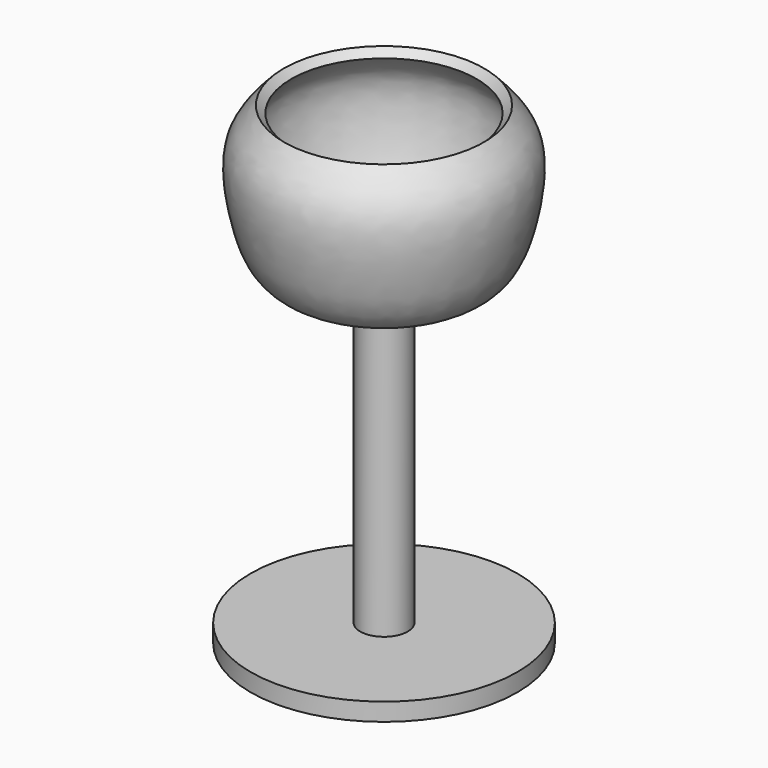
from build123d import *


# Not quite as in the source:
# - the dataset's text gives a spline's control points without its knots; the knots are read off the source's solid


with BuildPart() as f1:
    # F0 (on Front) → F1 (revolve)
    with BuildSketch(Plane.XZ):
        with BuildLine():
            Line((-33.3114092118, -56.5219796077), (-3.3958540803, -56.5219796077))
            Line((-3.3958540803, -56.5219796077), (-3.3958540803, -52.0700030029))
            Line((-3.3958540803, -52.0700030029), (-3.3958540803, 17.4802527591))
            add(Edge.make_bspline(
                [(-3.3958540803, 17.4802527591), (-3.3958541705, 17.9874718655), (-3.4894182694, 18.9850607329), (-3.9552971661, 20.3950614541), (-4.7364240353, 21.6166062828), (-5.730456479, 22.5691381333), (-6.824989545, 23.2653337421), (-7.9612562833, 23.7659449911), (-9.1199618827, 24.1286972097), (-10.6872079124, 24.4847423795), (-12.6794090241, 24.7690811344), (-15.057700209, 25.020810082), (-16.9353054891, 25.2572720748), (-18.3004868031, 25.5091381546), (-19.0782015912, 25.6983898999), (-19.6453651181, 25.8706576014), (-20.1689159088, 26.0552640278), (-21.0237206953, 26.4289307261), (-22.0986256248, 27.1000061621), (-23.2231720549, 28.1270764831), (-24.2169952979, 29.3842127548), (-25.0906025524, 30.8622732772), (-25.8487547346, 32.5336407625), (-26.499795979, 34.3600080021), (-27.0576108529, 36.2980435215), (-27.4605598647, 37.9723758628), (-27.7565000106, 39.3219389625), (-28.0298358786, 40.6563829608), (-28.3264085816, 42.2991263992), (-28.5978205058, 44.2112486043), (-28.7736609188, 46.0478262131), (-28.8439304516, 47.7907204674), (-28.800606266, 49.4213304286), (-28.638524177, 50.9204444011), (-28.356627804, 52.2715916344), (-27.957686014, 53.4579814442), (-27.4235612753, 54.5834120112), (-26.5464682961, 56.0262955132), (-25.1576533584, 57.7761666906), (-23.8232178448, 59.189069017), (-23.1318071392, 59.9196787403)],
                knots=[0, 0, 0, 0, 0.015625, 0.03125, 0.046875, 0.0625, 0.078125, 0.09375, 0.109375, 0.125, 0.15625, 0.1875, 0.21875, 0.234375, 0.25, 0.2578125, 0.265625, 0.28125, 0.3125, 0.34375, 0.375, 0.40625, 0.4375, 0.46875, 0.5, 0.53125, 0.546875, 0.5625, 0.59375, 0.625, 0.65625, 0.6875, 0.71875, 0.75, 0.78125, 0.8125, 0.84375, 0.875, 0.9375, 1, 1, 1, 1], degree=3))
            Line((-23.1318071392, 59.9196787403), (-24.9766670167, 61.6655573249))
            add(Edge.make_bspline(
                [(-5.9358540803, 17.4802523072), (-5.9358551295, 23.3771994857), (-24.558431826, 19.6331068284), (-30.7111519039, 37.8470595035), (-32.4281506403, 53.7832649491), (-27.2669888342, 59.2453874087), (-24.9766670167, 61.6655573249)],
                knots=[0, 0, 0, 0, 0.2626132896, 0.5343729414, 0.793047164, 1, 1, 1, 1], degree=3))
            Line((-5.9358540803, 17.4802523072), (-5.9358540803, -52.0700030029))
            Line((-5.9358540803, -52.0700030029), (-33.3114092118, -52.0700030029))
            Line((-33.3114092118, -52.0700030029), (-33.3114092118, -56.5219796077))
        make_face()
    revolve(axis=Axis((0, 0, 6.9780203923), (0, 0, -1)))


solid = f1.part
